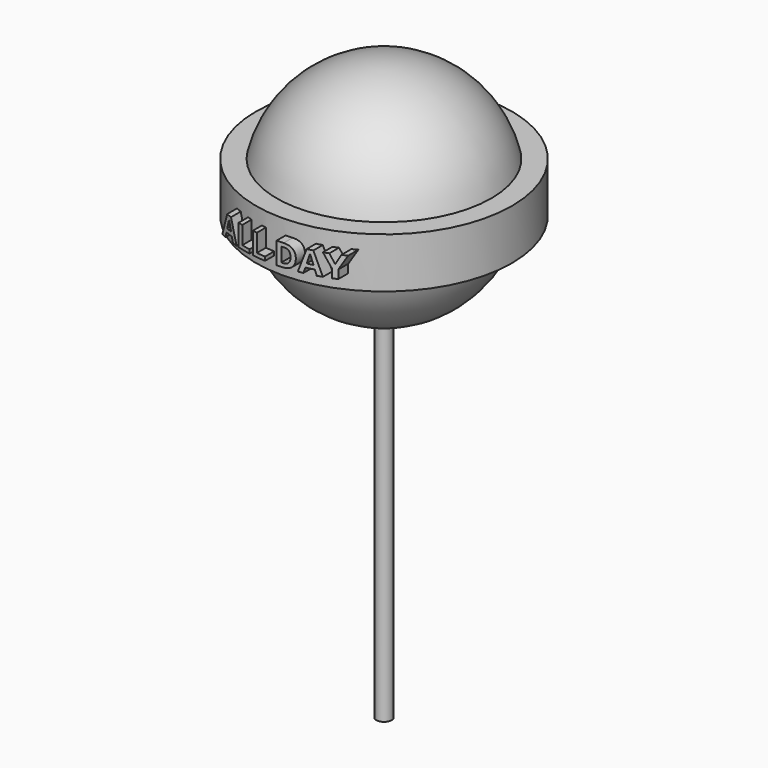
from build123d import *

# Parameters (mm, degrees)
F2_TEXT_SIZE = 6.8158027716
F3_DEPTH     = 45.72


# Not quite as in the source:
# - Text() gives the source's letters only with a copy of the font that has no kerning and outlines rounded to 1/6400 em; it was checked with that copy


with BuildPart() as f1:
    # F0 (on Front) → F1 (revolve)
    with BuildSketch(Plane.XZ):
        with BuildLine():
            Line((0, -16.0915702581), (0, -24.8246836828))
            ThreePointArc((0, -24.8246836828), (0.8554528759, -24.8099399501), (1.7098896205, -24.7657262651))
            Line((1.7098896205, -24.7657262651), (1.7098896205, -16.0915702581))
            Line((1.7098896205, -16.0915702581), (0, -16.0915702581))
        make_face()
        with BuildLine():
            ThreePointArc((1.7098896205, -24.7657262651), (0.8554528759, -24.8099399501), (0, -24.8246836828))
            Line((0, -24.8246836828), (0, -105.0746738911))
            Line((0, -105.0746738911), (1.7098896205, -105.0746738911))
            Line((1.7098896205, -105.0746738911), (1.7098896205, -24.7657262651))
        make_face()
        with BuildLine():
            Line((1.7098896205, -16.0915702581), (1.7098896205, -24.7657262651))
            ThreePointArc((1.7098896205, -24.7657262651), (16.0828444767, -18.9105006145), (24.1698625056, -5.6641562842))
            Line((24.1698625056, -5.6641562842), (0.4312911468, -5.6641562842))
            Line((0.4312911468, -5.6641562842), (0.4312911468, 5.6641562842))
            Line((0.4312911468, 5.6641562842), (24.1698625056, 5.6641562842))
            ThreePointArc((24.1698625056, 5.6641562842), (15.4216411556, 19.4534805117), (0, 24.8246836828))
            Line((0, 24.8246836828), (0, -16.0915702581))
            Line((0, -16.0915702581), (1.7098896205, -16.0915702581))
        make_face()
        with BuildLine():
            Line((0.4312911468, -5.6641562842), (24.1698625056, -5.6641562842))
            ThreePointArc((24.1698625056, -5.6641562842), (24.8246836828, 0), (24.1698625056, 5.6641562842))
            Line((24.1698625056, 5.6641562842), (0.4312911468, 5.6641562842))
            Line((0.4312911468, 5.6641562842), (0.4312911468, -5.6641562842))
        make_face()
        with BuildLine():
            ThreePointArc((24.1698625056, 5.6641562842), (24.8246836828, 0), (24.1698625056, -5.6641562842))
            Line((24.1698625056, -5.6641562842), (28.8096759468, -5.6641562842))
            Line((28.8096759468, -5.6641562842), (28.8096759468, 5.6641562842))
            Line((28.8096759468, 5.6641562842), (24.1698625056, 5.6641562842))
        make_face()
    revolve(axis=Axis((0, 0, 2.1533742547), (0, 0, -1)))

    # F2 (on Front) → F3 (join)
    with BuildSketch(Plane.XZ):
        with Locations((-13.9102791436, -2.4200372864)):
            Text('ALL DAY', F2_TEXT_SIZE, font='Open Sans', font_style=FontStyle.BOLD, text_align=(TextAlign.LEFT, TextAlign.BOTTOM))
    extrude(amount=F3_DEPTH)

    # F4 (on Front) → F6 (revolve, cut)
    with BuildSketch(Plane.XZ):
        Polygon((31.3496759468, -8.2041562842), (28.8096759468, -8.2041562842), (23.0203568935, -23.2014751369), (44.4879084826, -23.2014751369), (52.3418933153, 0), (42.9171174765, 18.5806194627), (19.0933663398, 18.5806194627), (28.8096759468, 8.2041562842), (31.3496759468, 8.2041562842), align=None)
    revolve(axis=Axis((0, 0, -1.4581568539), (0, 0, -1)), mode=Mode.SUBTRACT)


solid = f1.part
